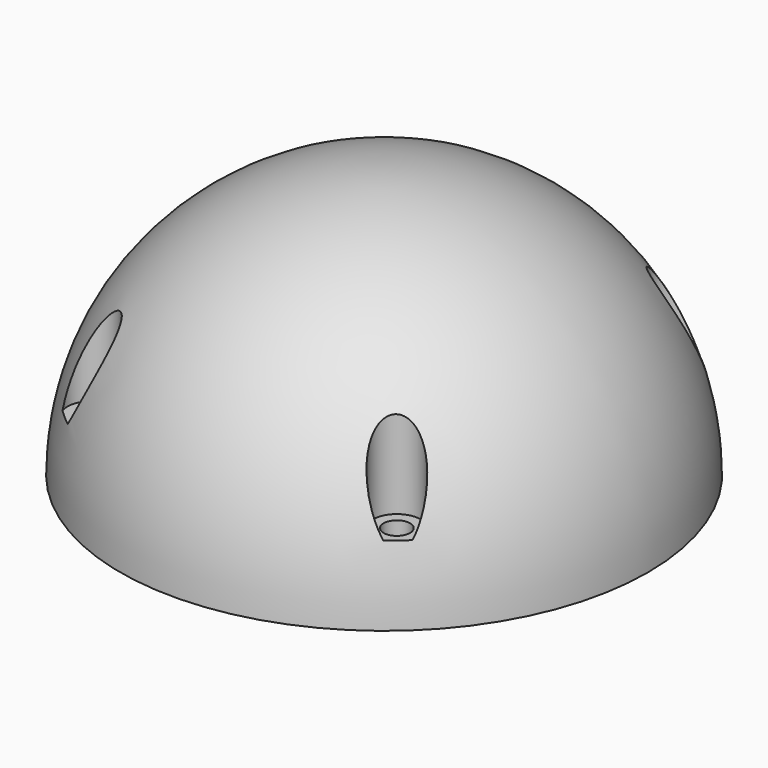
from build123d import *

# Parameters (mm, degrees)
F0_R           = 25
F1_DEPTH       = 25
F3_D           = 2.5
F3_CBORE_D     = 4.5
F3_CBORE_DEPTH = 18


# Not quite as in the source:
# - a fillet or chamfer that OpenCascade refuses, or shapes differently, is made with other operations: its cross-section is extruded or revolved along the edge and cut away or added


with BuildPart() as f1:
    # F0 (on Top) → F1 (new body)
    with BuildSketch(Plane.XY):
        Circle(F0_R)
    extrude(amount=F1_DEPTH)

    # F3 (through all)
    with Locations(Plane.XY.offset(25)):
        with Locations((14.4662138687, 16.5749406124), (14.4662138687, -16.5749406124), (-14.4662138687, -16.5749406124), (-14.4662138687, 16.5749406124)):
            CounterBoreHole(F3_D / 2, F3_CBORE_D / 2, F3_CBORE_DEPTH)

    # F4: fillet of radius 25 on 1 edges, made by hand

    # F4_s1 → F4_t2 (revolve, cut)
    with BuildSketch(Plane.XZ):
        with BuildLine():
            ThreePointArc((25, 0), (17.6776695297, 17.6776695297), (0, 25))
            Line((0, 25), (25, 25))
            Line((25, 25), (25, 0))
        make_face()
    revolve(axis=Axis((0, 0, 25), (0, 0, 1)), mode=Mode.SUBTRACT)


solid = f1.part
